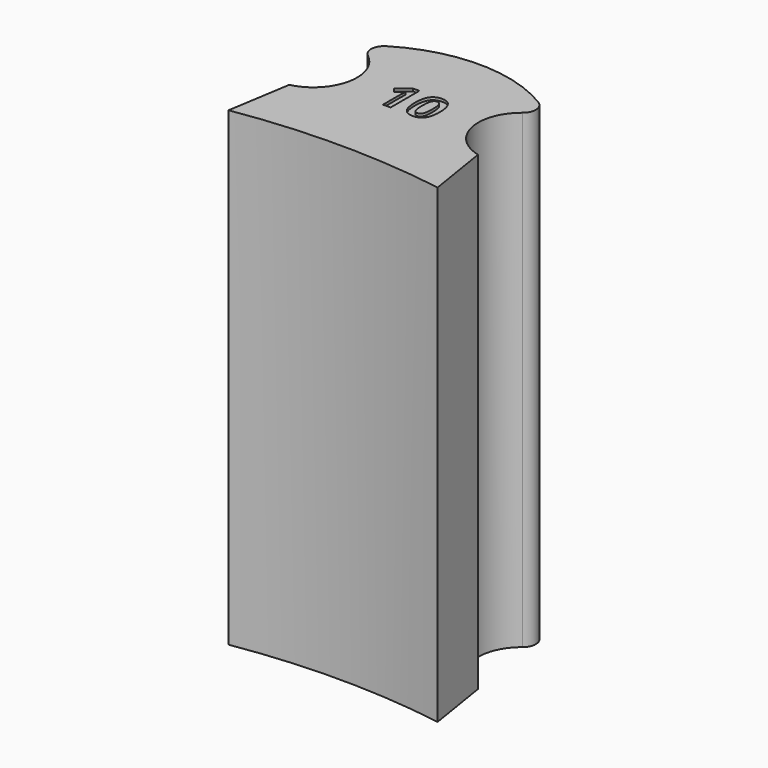
from build123d import *

# Parameters (mm, degrees)
F1_DEPTH     = 180
F2_TEXT_SIZE = 19.2989440014
F3_DEPTH     = 1


# Not quite as in the source:
# - Text() gives the source's letters only with a copy of the font that has no kerning and outlines rounded to 1/6400 em; it was checked with that copy


with BuildPart() as f1:
    # F0 (on Top) → F1 (new body)
    with BuildSketch(Plane.XY):
        with BuildLine():
            Line((3.8687128108, 24.1569802165), (0, 0))
            ThreePointArc((0, 0), (40, 3.1820662963), (80, 0))
            Line((80, 0), (76.1312871892, 24.1569802165))
            ThreePointArc((76.1312871892, 24.1569802165), (63.5975554576, 36.8458138953), (69.5972800683, 53.6417728094))
            ThreePointArc((69.5972800683, 53.6417728094), (71.4969098635, 57.8715436357), (69.1043731597, 61.843359684))
            ThreePointArc((69.1043731597, 61.843359684), (40, 70), (10.8956268403, 61.843359684))
            ThreePointArc((10.8956268403, 61.843359684), (8.5030901365, 57.8715436357), (10.4027199317, 53.6417728094))
            ThreePointArc((10.4027199317, 53.6417728094), (16.4024445424, 36.8458138953), (3.8687128108, 24.1569802165))
        make_face()
    extrude(amount=F1_DEPTH)

    # F2 (on face) → F3 (cut)
    with BuildSketch(Plane.XY.offset(180)):
        with Locations((28.7025791092, 31.6558778286)):
            Text('10', F2_TEXT_SIZE, font='Open Sans', font_style=FontStyle.BOLD, text_align=(TextAlign.LEFT, TextAlign.BOTTOM))
    extrude(amount=-F3_DEPTH, mode=Mode.SUBTRACT)


solid = f1.part
